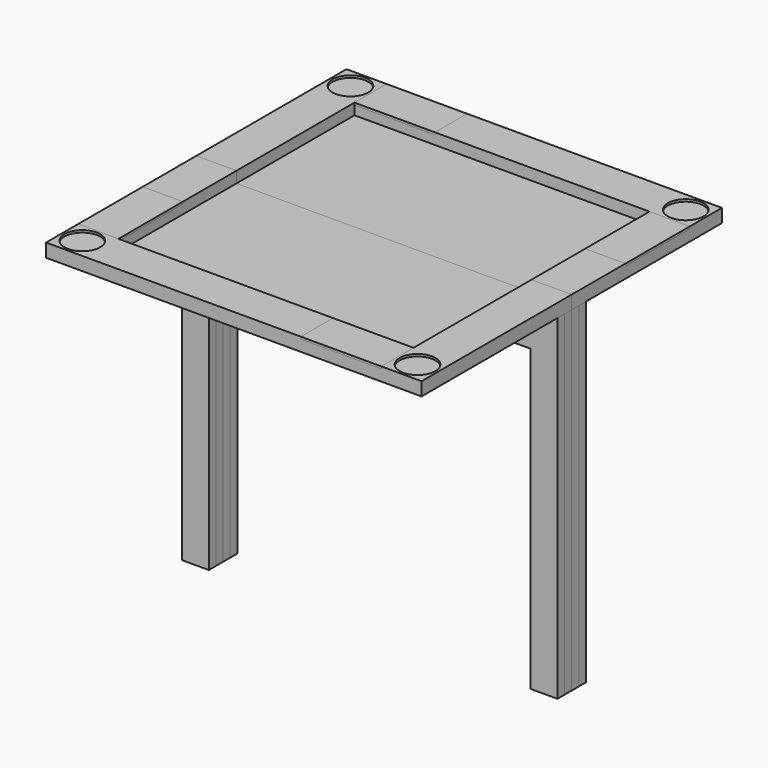
from build123d import *

# Parameters (mm, degrees)
F0_W      = 840
F0_H      = 5
F1_DEPTH  = 420
F2_DEPTH  = 420
F3_R      = 40
F3_W      = 90
F3_H      = 150
F3_H_2    = 180
F3_W_2    = 80
F3_H_3    = 170
F3_W_3    = 180
F3_H_4    = 90
F3_W_4    = 170
F3_H_5    = 80
F4_DEPTH  = 30
F3_W_5    = 80.0002463284
F5_DEPTH  = 30
F3_W_6    = 0.0002463284
F6_DEPTH  = 5
F11_DEPTH = 750
F10_W     = 420
F10_H     = 20
F12_DEPTH = 750
F13_DEPTH = 750
F14_W     = 720
F14_H     = 670
F15_DEPTH = 201


with BuildPart() as f1:
    # F0 (on Front) → F1 (new body)
    with BuildSketch(Plane.XZ):
        with Locations((0, -12.5)):
            Rectangle(F0_W, F0_H)
    extrude(amount=F1_DEPTH)

    # F3 (on face) → F5 (join)
    with BuildSketch(Plane(origin=(0, 0, -15), x_dir=(1, 0, 0), z_dir=(0, 0, -1))):
        with Locations((-375, 75)):
            Rectangle(F3_W, F3_H)
        Polygon((-330, 330), (150, 330), (150, 420), (-420, 420), (-420, 330), align=None)
        with Locations((-375.0001231642, 375)):
            Circle(F3_R, mode=Mode.SUBTRACT)
        Polygon((330, 330), (330, 0), (420, 0), (420, 420), (330, 420), align=None)
        with Locations((375, 375)):
            Circle(F3_R, mode=Mode.SUBTRACT)
        with Locations((-375.0001231642, 375)):
            Circle(F3_R)
        with Locations((375, 375)):
            Circle(F3_R)
        with Locations((-375, 240)):
            Rectangle(F3_W, F3_H_2)
        with Locations((-375.0001231642, 240)):
            Rectangle(F3_W_5, F3_H_3, mode=Mode.SUBTRACT)
        with Locations((240, 375)):
            Rectangle(F3_W_3, F3_H_4)
        with Locations((240, 375)):
            Rectangle(F3_W_4, F3_H_5, mode=Mode.SUBTRACT)
    extrude(amount=-F5_DEPTH)


with BuildPart() as f2:
    # F0 (on Front) → F2 (new body)
    with BuildSketch(Plane.XZ):
        with Locations((0, -12.5)):
            Rectangle(F0_W, F0_H)
    extrude(amount=-F2_DEPTH)

    # F3 (on face) → F4 (join)
    with BuildSketch(Plane(origin=(0, 0, -15), x_dir=(1, 0, 0), z_dir=(0, 0, -1))):
        Polygon((420, -330), (330, -330), (-150, -330), (-150, -420), (420, -420), align=None)
        with Locations((375, -375)):
            Circle(F3_R, mode=Mode.SUBTRACT)
        Polygon((-330, -420), (-330, -330), (-330, 0), (-420, 0), (-420, -420), align=None)
        with Locations((-375.0001231642, -375)):
            Circle(F3_R, mode=Mode.SUBTRACT)
        with Locations((375, -75)):
            Rectangle(F3_W, F3_H)
        with Locations((375, -240)):
            Rectangle(F3_W, F3_H_2)
        with Locations((375, -240)):
            Rectangle(F3_W_2, F3_H_3, mode=Mode.SUBTRACT)
        with Locations((-240, -375)):
            Rectangle(F3_W_3, F3_H_4)
        with Locations((-240, -375)):
            Rectangle(F3_W_4, F3_H_5, mode=Mode.SUBTRACT)
        with Locations((-375.0001231642, -375)):
            Circle(F3_R)
        with Locations((375, -375)):
            Circle(F3_R)
    extrude(amount=-F4_DEPTH)


with BuildPart() as f6:
    # F3 (on face) → F6 (new body)
    with BuildSketch(Plane(origin=(0, 0, -15), x_dir=(1, 0, 0), z_dir=(0, 0, -1))):
        with Locations((-375, 240)):
            Rectangle(F3_W, F3_H_2)
        with Locations((-375.0001231642, 240)):
            Rectangle(F3_W_5, F3_H_3, mode=Mode.SUBTRACT)
        with Locations((-375.0001231642, 240)):
            Rectangle(F3_W_5, F3_H_3)
        with Locations((-420.0001231642, 240)):
            Rectangle(F3_W_6, F3_H_2)
    extrude(amount=-F6_DEPTH)


with BuildPart() as f6b:
    # F3 (on face) → F6, piece 2 (new body)
    with BuildSketch(Plane(origin=(0, 0, -15), x_dir=(1, 0, 0), z_dir=(0, 0, -1))):
        with Locations((240, 375)):
            Rectangle(F3_W_3, F3_H_4)
        with Locations((240, 375)):
            Rectangle(F3_W_4, F3_H_5, mode=Mode.SUBTRACT)
        with Locations((240, 375)):
            Rectangle(F3_W_4, F3_H_5)
    extrude(amount=-F6_DEPTH)


with BuildPart() as f6c:
    # F3 (on face) → F6, piece 3 (new body)
    with BuildSketch(Plane(origin=(0, 0, -15), x_dir=(1, 0, 0), z_dir=(0, 0, -1))):
        with Locations((375, -240)):
            Rectangle(F3_W, F3_H_2)
        with Locations((375, -240)):
            Rectangle(F3_W_2, F3_H_3, mode=Mode.SUBTRACT)
        with Locations((375, -240)):
            Rectangle(F3_W_2, F3_H_3)
    extrude(amount=-F6_DEPTH)


with BuildPart() as f6d:
    # F3 (on face) → F6, piece 4 (new body)
    with BuildSketch(Plane(origin=(0, 0, -15), x_dir=(1, 0, 0), z_dir=(0, 0, -1))):
        with Locations((-240, -375)):
            Rectangle(F3_W_3, F3_H_4)
        with Locations((-240, -375)):
            Rectangle(F3_W_4, F3_H_5, mode=Mode.SUBTRACT)
        with Locations((-240, -375)):
            Rectangle(F3_W_4, F3_H_5)
    extrude(amount=-F6_DEPTH)


with BuildPart() as f6e:
    # F3 (on face) → F6, piece 5 (new body)
    with BuildSketch(Plane(origin=(0, 0, -15), x_dir=(1, 0, 0), z_dir=(0, 0, -1))):
        with Locations((-375.0001231642, 375)):
            Circle(F3_R)
    extrude(amount=-F6_DEPTH)


with BuildPart() as f6f:
    # F3 (on face) → F6, piece 6 (new body)
    with BuildSketch(Plane(origin=(0, 0, -15), x_dir=(1, 0, 0), z_dir=(0, 0, -1))):
        with Locations((-375.0001231642, -375)):
            Circle(F3_R)
    extrude(amount=-F6_DEPTH)


with BuildPart() as f6g:
    # F3 (on face) → F6, piece 7 (new body)
    with BuildSketch(Plane(origin=(0, 0, -15), x_dir=(1, 0, 0), z_dir=(0, 0, -1))):
        with Locations((375, -375)):
            Circle(F3_R)
    extrude(amount=-F6_DEPTH)


with BuildPart() as f6h:
    # F3 (on face) → F6, piece 8 (new body)
    with BuildSketch(Plane(origin=(0, 0, -15), x_dir=(1, 0, 0), z_dir=(0, 0, -1))):
        with Locations((375, 375)):
            Circle(F3_R)
    extrude(amount=-F6_DEPTH)


with BuildPart() as f6d_1:
    # F7: moved
    add(f6d.part.moved(Location((0, 0, 25))))


with BuildPart() as f6_1:
    # F7: moved
    add(f6.part.moved(Location((0, 0, 25))))


with BuildPart() as f6c_1:
    # F7: moved
    add(f6c.part.moved(Location((0, 0, 25))))


with BuildPart() as f6b_1:
    # F7: moved
    add(f6b.part.moved(Location((0, 0, 25))))


with BuildPart() as f6f_1:
    # F7: moved
    add(f6f.part.moved(Location((0, 0, 25))))


with BuildPart() as f6e_1:
    # F7: moved
    add(f6e.part.moved(Location((0, 0, 25))))


with BuildPart() as f6h_1:
    # F7: moved
    add(f6h.part.moved(Location((0, 0, 25))))


with BuildPart() as f6g_1:
    # F7: moved
    add(f6g.part.moved(Location((0, 0, 25))))


with BuildPart() as f2_1:
    add(f2.part)

    # F8: cut F6d, F6c, F6b, F6
    add(f6d_1.part, mode=Mode.SUBTRACT)
    add(f6c_1.part, mode=Mode.SUBTRACT)
    add(f6b_1.part, mode=Mode.SUBTRACT)
    add(f6_1.part, mode=Mode.SUBTRACT)

    # F9: cut F6g, F6f, F6e, F6h
    add(f6g_1.part, mode=Mode.SUBTRACT)
    add(f6f_1.part, mode=Mode.SUBTRACT)
    add(f6e_1.part, mode=Mode.SUBTRACT)
    add(f6h_1.part, mode=Mode.SUBTRACT)


with BuildPart() as f1_1:
    add(f1.part)

    # F8: cut F6d, F6c, F6b, F6
    add(f6d_1.part, mode=Mode.SUBTRACT)
    add(f6c_1.part, mode=Mode.SUBTRACT)
    add(f6b_1.part, mode=Mode.SUBTRACT)
    add(f6_1.part, mode=Mode.SUBTRACT)

    # F9: cut F6g, F6f, F6e, F6h
    add(f6g_1.part, mode=Mode.SUBTRACT)
    add(f6f_1.part, mode=Mode.SUBTRACT)
    add(f6e_1.part, mode=Mode.SUBTRACT)
    add(f6h_1.part, mode=Mode.SUBTRACT)


with BuildPart() as f11:
    # F10 (on face) → F11 (new body)
    with BuildSketch(Plane(origin=(0, 0, -15), x_dir=(1, 0, 0), z_dir=(0, 0, -1))):
        Polygon((-420, 40), (-420, 20), (0, 20), (420, 20), (420, 40), align=None)
    extrude(amount=F11_DEPTH)


with BuildPart() as f11b:
    # F10 (on face) → F11, piece 2 (new body)
    with BuildSketch(Plane(origin=(0, 0, -15), x_dir=(1, 0, 0), z_dir=(0, 0, -1))):
        Polygon((0, -20), (-420, -20), (-420, -40), (420, -40), (420, -20), align=None)
    extrude(amount=F11_DEPTH)


with BuildPart() as f12:
    # F10 (on face) → F12 (new body, through all)
    with BuildSketch(Plane(origin=(0, 0, -15), x_dir=(1, 0, 0), z_dir=(0, 0, -1))):
        with Locations((-210, 10)):
            Rectangle(F10_W, F10_H)
    extrude(amount=F12_DEPTH)


with BuildPart() as f12b:
    # F10 (on face) → F12, piece 2 (new body, through all)
    with BuildSketch(Plane(origin=(0, 0, -15), x_dir=(1, 0, 0), z_dir=(0, 0, -1))):
        with Locations((210, -10)):
            Rectangle(F10_W, F10_H)
    extrude(amount=F12_DEPTH)


with BuildPart() as f13:
    # F10 (on face) → F13 (new body, through all)
    with BuildSketch(Plane(origin=(0, 0, -15), x_dir=(1, 0, 0), z_dir=(0, 0, -1))):
        with Locations((210, 10)):
            Rectangle(F10_W, F10_H)
    extrude(amount=F13_DEPTH)


with BuildPart() as f13b:
    # F10 (on face) → F13, piece 2 (new body, through all)
    with BuildSketch(Plane(origin=(0, 0, -15), x_dir=(1, 0, 0), z_dir=(0, 0, -1))):
        with Locations((-210, -10)):
            Rectangle(F10_W, F10_H)
    extrude(amount=F13_DEPTH)


with BuildPart() as f15_tool:
    # F14 (on face) → F15 (new body)
    with BuildSketch(Plane.XZ.offset(40)):
        with Locations((0, -430)):
            Rectangle(F14_W, F14_H)
    extrude(amount=-F15_DEPTH)


with BuildPart() as f11_1:
    add(f11.part)

    # F15: cut by f15_tool
    add(f15_tool.part, mode=Mode.SUBTRACT)


with BuildPart() as f11b_1:
    add(f11b.part)

    # F15: cut by f15_tool
    add(f15_tool.part, mode=Mode.SUBTRACT)


with BuildPart() as f12_1:
    add(f12.part)

    # F15: cut by f15_tool
    add(f15_tool.part, mode=Mode.SUBTRACT)


with BuildPart() as f12b_1:
    add(f12b.part)

    # F15: cut by f15_tool
    add(f15_tool.part, mode=Mode.SUBTRACT)


with BuildPart() as f13_1:
    add(f13.part)

    # F15: cut by f15_tool
    add(f15_tool.part, mode=Mode.SUBTRACT)


with BuildPart() as f13b_1:
    add(f13b.part)

    # F15: cut by f15_tool
    add(f15_tool.part, mode=Mode.SUBTRACT)


solid = Compound([f6d_1.part, f6_1.part, f6c_1.part, f6b_1.part, f2_1.part, f1_1.part, f11_1.part, f11b_1.part, f12_1.part, f12b_1.part, f13_1.part, f13b_1.part])
